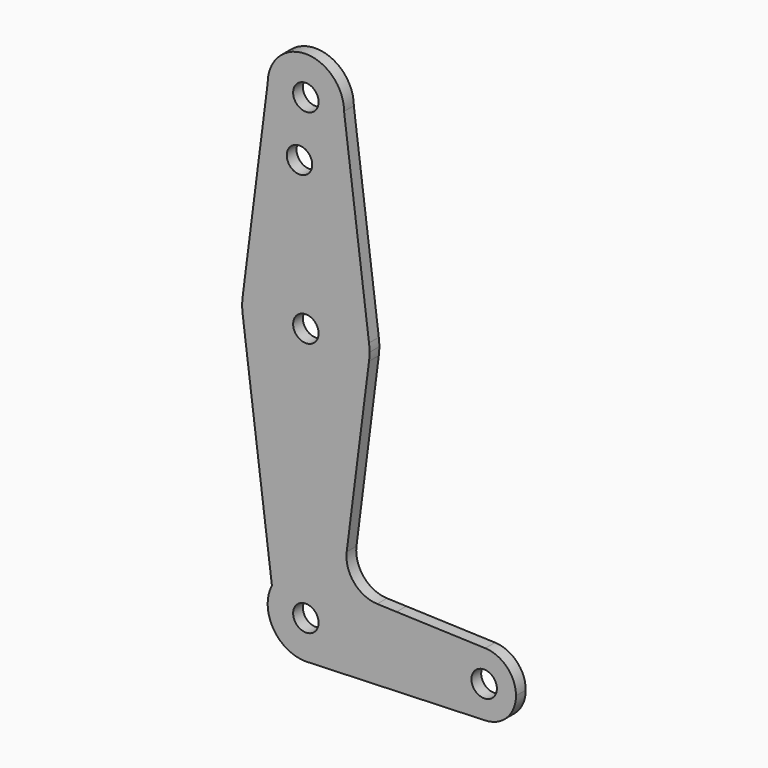
from build123d import *

# Parameters (mm, degrees)
F0_R     = 3.175
F1_DEPTH = 3.048


# Not quite as in the source:
# - ends of sketch curves that miss each other by under 0.0002 mm in the source are joined


with BuildPart() as f1:
    # F0 (on Front) → F1 (new body)
    with BuildSketch(Plane.XZ):
        with BuildLine():
            ThreePointArc((-9.525, 114.3), (0, 104.775), (9.525, 114.3))
            ThreePointArc((9.525, 114.3), (0, 123.825), (-9.525, 114.3))
        make_face()
        with Locations((0, 114.3)):
            Circle(F0_R, mode=Mode.SUBTRACT)
        with BuildLine():
            Line((15.7474569047, 65.5082893304), (9.525, 114.3))
            ThreePointArc((9.525, 114.3), (0, 104.775), (-9.525, 114.3))
            Line((-9.525, 114.3), (-15.7474569047, 65.5082893304))
            ThreePointArc((-15.7474569047, 65.5082893304), (0, 79.375), (15.7474569047, 65.5082893304))
        make_face()
        with Locations((-1.5875, 100.0252)):
            Circle(F0_R, mode=Mode.SUBTRACT)
        with BuildLine():
            ThreePointArc((15.875, 63.5), (15.8430821396, 64.5061676396), (15.7474569047, 65.5082893304))
            ThreePointArc((15.7474569047, 65.5082893304), (0, 79.375), (-15.7474569047, 65.5082893304))
            ThreePointArc((-15.7474569047, 65.5082893304), (-15.875, 63.5), (-15.7474569047, 61.4917106696))
            ThreePointArc((-15.7474569047, 61.4917106696), (0, 47.625), (15.7474569047, 61.4917106696))
            ThreePointArc((15.7474569047, 61.4917106696), (15.8430821396, 62.4938323604), (15.875, 63.5))
        make_face()
        with Locations((0, 63.5)):
            Circle(F0_R, mode=Mode.SUBTRACT)
        with BuildLine():
            ThreePointArc((15.7474569047, 61.4917106696), (0, 47.625), (-15.7474569047, 61.4917106696))
            Line((-15.7474569047, 61.4917106696), (-8.4628069595, 4.371100933))
            ThreePointArc((-8.4628069595, 4.371100933), (2.2491541422, 9.2556431783), (9.525, 0))
            ThreePointArc((9.525, 0), (6.9705567315, -6.4912990883), (0.6773435479, -9.500885786))
            Line((0.6773435479, -9.500885786), (44.7324052746, -7.9324746146))
            ThreePointArc((44.7324052746, -7.9324746146), (36.5125, 0), (44.7324052746, 7.9324746146))
            Line((44.7324052746, 7.9324746146), (22.606619146, 8.7201782014))
            Line((22.606619146, 8.7201782014), (17.7823482037, 8.8932352229))
            ThreePointArc((17.7823482037, 8.8932352229), (12.00790709, 11.6916015121), (10.1808634842, 17.8427750365))
            Line((10.1808634842, 17.8427750365), (10.1810293195, 17.844076245))
            Line((10.1810293195, 17.844076245), (15.7474569047, 61.4917106696))
        make_face()
        with BuildLine():
            ThreePointArc((9.525, 0), (2.2491541422, 9.2556431783), (-8.4628069595, 4.371100933))
            ThreePointArc((-8.4628069595, 4.371100933), (-8.1351202015, -4.9543359097), (0, -9.525))
            Line((0, -9.525), (0.6773435479, -9.500885786))
            ThreePointArc((0.6773435479, -9.500885786), (6.9705567315, -6.4912990883), (9.525, 0))
        make_face()
        Circle(F0_R, mode=Mode.SUBTRACT)
        with BuildLine():
            Line((0.6773435479, -9.500885786), (0, -9.525))
            ThreePointArc((0, -9.525), (0.3388863295, -9.5189695375), (0.6773435479, -9.500885786))
        make_face()
        with BuildLine():
            ThreePointArc((44.7324052746, 7.9324746146), (36.5125, 0), (44.7324052746, -7.9324746146))
            ThreePointArc((44.7324052746, -7.9324746146), (50.1616327839, -5.5119104847), (52.3875, 0))
            ThreePointArc((52.3875, 0), (50.1616327839, 5.5119104847), (44.7324052746, 7.9324746146))
        make_face()
        with Locations((44.45, 0)):
            Circle(F0_R, mode=Mode.SUBTRACT)
    extrude(amount=F1_DEPTH)


solid = f1.part
